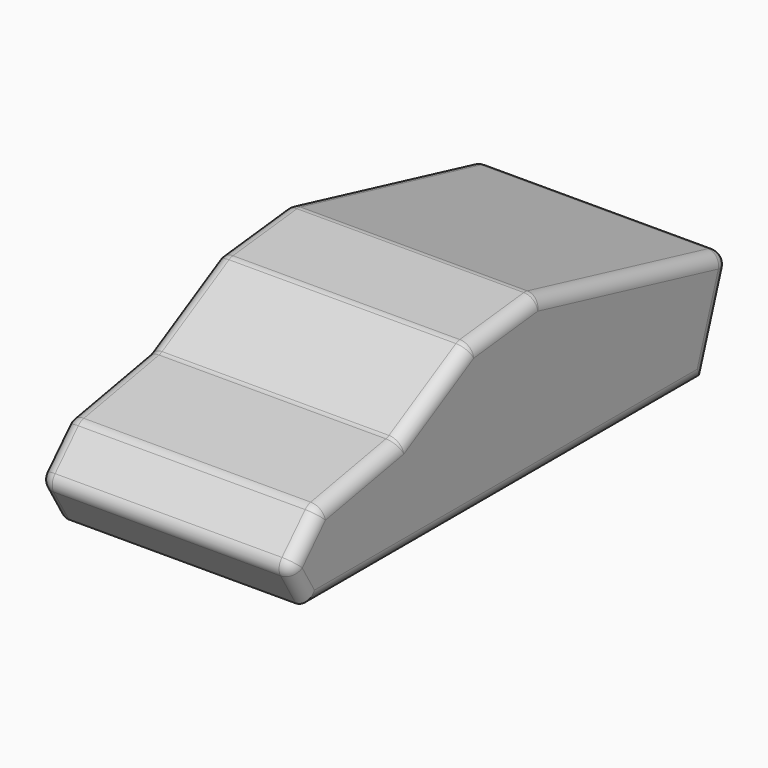
from build123d import *

# Parameters (mm, degrees)
F1_DEPTH     = 99.822
F2_R         = 5.08
F3_R         = 5.08
F4_F1_R      = 5.08
F4_T2_DEPTH  = 89.662
F4_T7_DEPTH  = 5.1816
F4_T13_DEPTH = 5.1816
F4_T19_DEPTH = 5.1816
F4_T25_DEPTH = 5.1816
F4_T31_DEPTH = 5.1816
F4_T37_DEPTH = 5.1816
F4_T43_DEPTH = 5.1816
F4_T49_DEPTH = 5.1816
F4_T55_DEPTH = 5.1816
F4_T61_DEPTH = 5.1816


# Not quite as in the source:
# - a fillet or chamfer that OpenCascade refuses, or shapes differently, is made with other operations: its cross-section is extruded or revolved along the edge and cut away or added


with BuildPart() as f1:
    # F0 (on Right) → F1 (new body)
    with BuildSketch(Plane.YZ):
        Polygon((-82.3224335909, 15.9557517618), (-72.8414729238, 0), (122.7899119258, 0), (136.201992631, 39.3112748861), (40.6987294555, 62.4355487525), (7.1685267612, 58.7356649339), (-27.5178905576, 39.3112748861), (-67.0604035258, 31.9115035236), align=None)
    extrude(amount=F1_DEPTH)

    # F2
    f2_edges = [f1.edges().sort_by_distance(p)[0] for p in [
        (99.822, -47.289147, 35.611389),
        (99.822, -74.691419, 23.933628),
        (99.822, -77.581953, 7.977876),
        (99.822, 24.97422, 0),
        (99.822, 129.495952, 19.655637),
        (99.822, 88.450361, 50.873412),
        (99.822, 23.933628, 60.585607),
        (99.822, -10.174682, 49.02347),
    ]]
    fillet(f2_edges, radius=F2_R)

    # F3
    f3_edges = [f1.edges().sort_by_distance(p)[0] for p in [
        (0, -47.289147, 35.611389),
        (0, -74.691419, 23.933628),
        (0, -77.581953, 7.977876),
        (0, 24.97422, 0),
        (0, 129.495952, 19.655637),
        (0, 88.450361, 50.873412),
        (0, 23.933628, 60.585607),
        (0, -10.174682, 49.02347),
    ]]
    fillet(f3_edges, radius=F3_R)

    # F4: fillet of radius 5.08 on 8 edges, made by hand

    # F4_f1
    f4_f1_edges = [f1.edges().sort_by_distance(p)[0] for p in [
        (49.911, -27.5178905576, 39.3112748861),
        (1.4878975516, -27.0040618743, 37.8937040228),
        (98.3341025696, -27.0040618325, 37.8937039074),
    ]]
    fillet(f4_f1_edges, radius=F4_F1_R)

    # F4_s3 → F4_t2 (cut)
    with BuildSketch(Plane.YZ.offset(5.08)):
        with BuildLine():
            ThreePointArc((-65.453685614, 32.2121759973), (-66.9382582043, 31.6859414336), (-68.1902824988, 30.7302669295))
            Line((-68.1902824988, 30.7302669295), (-68.2637028962, 30.8004951663))
            Line((-68.2637028962, 30.8004951663), (-67.1112263438, 32.0053564923))
            Line((-67.1112263438, 32.0053564923), (-65.4723740737, 32.3120424155))
            Line((-65.4723740737, 32.3120424155), (-65.453685614, 32.2121759973))
        make_face()
        with BuildLine():
            ThreePointArc((-79.6549091873, 18.7445260612), (-81.0311938802, 15.8085415748), (-80.3510820874, 12.6381137788))
            Line((-80.3510820874, 12.6381137788), (-80.4384259429, 12.5862137699))
            Line((-80.4384259429, 12.5862137699), (-82.4492044764, 15.9702045126))
            Line((-82.4492044764, 15.9702045126), (-79.7283295848, 18.8147542979))
            Line((-79.7283295848, 18.8147542979), (-79.6549091873, 18.7445260612))
        make_face()
        with BuildLine():
            ThreePointArc((6.2686920086, 58.2317575672), (7.2001593092, 58.6369802666), (8.1936269176, 58.8487794151))
            Line((8.1936269176, 58.8487794151), (8.1824835206, 58.9497664672))
            Line((8.1824835206, 58.9497664672), (7.1368813611, 58.8343896965))
            Line((7.1368813611, 58.8343896965), (6.2190499134, 58.3204041823))
            Line((6.2190499134, 58.3204041823), (6.2686920086, 58.2317575672))
        make_face()
        with BuildLine():
            ThreePointArc((39.8125749839, 62.3377662065), (40.6937772364, 62.3580687153), (41.5652241428, 62.2257437701))
            Line((41.5652241428, 62.2257437701), (41.589133729, 62.3244903735))
            Line((41.589133729, 62.3244903735), (40.7053091479, 62.5384914556))
            Line((40.7053091479, 62.5384914556), (39.8014315869, 62.4387532586))
            Line((39.8014315869, 62.4387532586), (39.8125749839, 62.3377662065))
        make_face()
        with BuildLine():
            ThreePointArc((130.792336403, 40.6211188431), (134.0495526612, 38.1291725243), (134.4047361425, 34.0434536277))
            Line((134.4047361425, 34.0434536277), (134.5008937235, 34.0106469268))
            Line((134.5008937235, 34.0106469268), (136.3340953417, 39.3838246104))
            Line((136.3340953417, 39.3838246104), (130.8162459892, 40.7198654465))
            Line((130.8162459892, 40.7198654465), (130.792336403, 40.6211188431))
        make_face()
    extrude(amount=F4_T2_DEPTH, mode=Mode.SUBTRACT)


with BuildPart() as f4_tool5:
    # F4_s6 → F4_t7 (new body)
    with BuildSketch(Plane.YZ.offset(5.08)):
        Polygon((129.5968570941, 35.6837886716), (130.8162459892, 40.7198654465), (136.3340953417, 39.3838246104), (134.5008937235, 34.0106469268), align=None)
    extrude(amount=-F4_T7_DEPTH)

    # F4_s8 → F4_t9 (revolve, cut)
    with BuildSketch(Plane(origin=(5.08, 129.5968570941, 35.6837886716), x_dir=(0, -0.8765148754, -0.4813747742), z_dir=(0, 0.4813747742, -0.8765148754))):
        with BuildLine():
            ThreePointArc((0, -5.08), (5.08, 0), (0, 5.08))
            Line((0, 5.08), (0, -5.08))
        make_face()
    revolve(axis=Axis((5.08, 129.5968570941, 35.6837886716), (-1, 0, 0)), mode=Mode.SUBTRACT)


with BuildPart() as f1_1:
    add(f1.part)

    # F4_t4: cut F4_tool5
    add(f4_tool5.part, mode=Mode.SUBTRACT)


with BuildPart() as f4_tool11:
    # F4_s12 → F4_t13 (new body)
    with BuildSketch(Plane.YZ.offset(94.742)):
        Polygon((129.5968570941, 35.6837886716), (130.8162459892, 40.7198654465), (136.3340953417, 39.3838246104), (134.5008937235, 34.0106469268), align=None)
    extrude(amount=F4_T13_DEPTH)

    # F4_s14 → F4_t15 (revolve, cut)
    with BuildSketch(Plane(origin=(94.742, 129.5968570941, 35.6837886716), x_dir=(0, -0.8765148754, -0.4813747742), z_dir=(0, -0.4813747742, 0.8765148754))):
        with BuildLine():
            ThreePointArc((0, -5.08), (5.08, 0), (0, 5.08))
            Line((0, 5.08), (0, -5.08))
        make_face()
    revolve(axis=Axis((94.742, 129.5968570941, 35.6837886716), (1, 0, 0)), mode=Mode.SUBTRACT)


with BuildPart() as f1_2:
    add(f1_1.part)

    # F4_t10: cut F4_tool11
    add(f4_tool11.part, mode=Mode.SUBTRACT)


with BuildPart() as f4_tool17:
    # F4_s18 → F4_t19 (new body)
    with BuildSketch(Plane.YZ.offset(5.08)):
        Polygon((40.369744834, 57.2884135986), (39.8014315869, 62.4387532586), (40.7053091479, 62.5384914556), (41.589133729, 62.3244903735), align=None)
    extrude(amount=-F4_T19_DEPTH)

    # F4_s20 → F4_t21 (revolve, cut)
    with BuildSketch(Plane(origin=(5.08, 40.369744834, 57.2884135986), x_dir=(0, -0.063785906, -0.9979636056), z_dir=(0, 0.9979636056, -0.063785906))):
        with BuildLine():
            ThreePointArc((0, -5.08), (5.08, 0), (0, 5.08))
            Line((0, 5.08), (0, -5.08))
        make_face()
    revolve(axis=Axis((5.08, 40.369744834, 57.2884135986), (-1, 0, 0)), mode=Mode.SUBTRACT)


with BuildPart() as f1_3:
    add(f1_2.part)

    # F4_t16: cut F4_tool17
    add(f4_tool17.part, mode=Mode.SUBTRACT)


with BuildPart() as f4_tool23:
    # F4_s24 → F4_t25 (new body)
    with BuildSketch(Plane.YZ.offset(94.742)):
        Polygon((40.369744834, 57.2884135986), (39.8014315869, 62.4387532586), (40.7053091479, 62.5384914556), (41.589133729, 62.3244903735), align=None)
    extrude(amount=F4_T25_DEPTH)

    # F4_s26 → F4_t27 (revolve, cut)
    with BuildSketch(Plane(origin=(94.742, 40.369744834, 57.2884135986), x_dir=(0, -0.063785906, -0.9979636056), z_dir=(0, -0.9979636056, 0.063785906))):
        with BuildLine():
            ThreePointArc((0, -5.08), (5.08, 0), (0, 5.08))
            Line((0, 5.08), (0, -5.08))
        make_face()
    revolve(axis=Axis((94.742, 40.369744834, 57.2884135986), (1, 0, 0)), mode=Mode.SUBTRACT)


with BuildPart() as f1_4:
    add(f1_3.part)

    # F4_t22: cut F4_tool23
    add(f4_tool23.part, mode=Mode.SUBTRACT)


with BuildPart() as f4_tool29:
    # F4_s30 → F4_t31 (new body)
    with BuildSketch(Plane.YZ.offset(5.08)):
        Polygon((8.7507967676, 53.7994268073), (6.2190499134, 58.3204041823), (7.1368813611, 58.8343896965), (8.1824835206, 58.9497664672), align=None)
    extrude(amount=-F4_T31_DEPTH)

    # F4_s32 → F4_t33 (revolve, cut)
    with BuildSketch(Plane(origin=(5.08, 8.7507967676, 53.7994268073), x_dir=(0, 0.3052435942, -0.952274303), z_dir=(0, 0.952274303, 0.3052435942))):
        with BuildLine():
            ThreePointArc((0, -5.08), (5.08, 0), (0, 5.08))
            Line((0, 5.08), (0, -5.08))
        make_face()
    revolve(axis=Axis((5.08, 8.7507967676, 53.7994268073), (-1, 0, 0)), mode=Mode.SUBTRACT)


with BuildPart() as f1_5:
    add(f1_4.part)

    # F4_t28: cut F4_tool29
    add(f4_tool29.part, mode=Mode.SUBTRACT)


with BuildPart() as f4_tool35:
    # F4_s36 → F4_t37 (new body)
    with BuildSketch(Plane.YZ.offset(94.742)):
        Polygon((8.7507967676, 53.7994268073), (6.2190499134, 58.3204041823), (7.1368813611, 58.8343896965), (8.1824835206, 58.9497664672), align=None)
    extrude(amount=F4_T37_DEPTH)

    # F4_s38 → F4_t39 (revolve, cut)
    with BuildSketch(Plane(origin=(94.742, 8.7507967676, 53.7994268073), x_dir=(0, 0.3052435942, -0.952274303), z_dir=(0, -0.952274303, -0.3052435942))):
        with BuildLine():
            ThreePointArc((0, -5.08), (5.08, 0), (0, 5.08))
            Line((0, 5.08), (0, -5.08))
        make_face()
    revolve(axis=Axis((94.742, 8.7507967676, 53.7994268073), (1, 0, 0)), mode=Mode.SUBTRACT)


with BuildPart() as f1_6:
    add(f1_5.part)

    # F4_t34: cut F4_tool35
    add(f4_tool35.part, mode=Mode.SUBTRACT)


with BuildPart() as f4_tool41:
    # F4_s42 → F4_t43 (new body)
    with BuildSketch(Plane.YZ.offset(5.08)):
        Polygon((-75.9838893162, 15.2331142218), (-79.7283295848, 18.8147542979), (-82.4492044764, 15.9702045126), (-80.4384259429, 12.5862137699), align=None)
    extrude(amount=-F4_T43_DEPTH)

    # F4_s44 → F4_t45 (revolve, cut)
    with BuildSketch(Plane(origin=(5.08, -75.9838893162, 15.2331142218), x_dir=(0, 0.9935638905, -0.113273101), z_dir=(0, 0.113273101, 0.9935638905))):
        with BuildLine():
            ThreePointArc((0, -5.08), (5.08, 0), (0, 5.08))
            Line((0, 5.08), (0, -5.08))
        make_face()
    revolve(axis=Axis((5.08, -75.9838893162, 15.2331142218), (-1, 0, 0)), mode=Mode.SUBTRACT)


with BuildPart() as f1_7:
    add(f1_6.part)

    # F4_t40: cut F4_tool41
    add(f4_tool41.part, mode=Mode.SUBTRACT)


with BuildPart() as f4_tool47:
    # F4_s48 → F4_t49 (new body)
    with BuildSketch(Plane.YZ.offset(94.742)):
        Polygon((-75.9838893162, 15.2331142218), (-79.7283295848, 18.8147542979), (-82.4492044764, 15.9702045126), (-80.4384259429, 12.5862137699), align=None)
    extrude(amount=F4_T49_DEPTH)

    # F4_s50 → F4_t51 (revolve, cut)
    with BuildSketch(Plane(origin=(94.742, -75.9838893162, 15.2331142218), x_dir=(0, 0.9935638905, -0.113273101), z_dir=(0, -0.113273101, -0.9935638905))):
        with BuildLine():
            ThreePointArc((0, -5.08), (5.08, 0), (0, 5.08))
            Line((0, 5.08), (0, -5.08))
        make_face()
    revolve(axis=Axis((94.742, -75.9838893162, 15.2331142218), (1, 0, 0)), mode=Mode.SUBTRACT)


with BuildPart() as f1_8:
    add(f1_7.part)

    # F4_t46: cut F4_tool47
    add(f4_tool47.part, mode=Mode.SUBTRACT)


with BuildPart() as f4_tool53:
    # F4_s54 → F4_t55 (new body)
    with BuildSketch(Plane.YZ.offset(5.08)):
        Polygon((-64.5192626277, 27.2188550901), (-65.4723740737, 32.3120424155), (-67.1112263438, 32.0053564923), (-68.2637028962, 30.8004951663), align=None)
    extrude(amount=-F4_T55_DEPTH)

    # F4_s56 → F4_t57 (revolve, cut)
    with BuildSketch(Plane(origin=(5.08, -64.5192626277, 27.2188550901), x_dir=(0, 0.4761802316, -0.8793477054), z_dir=(0, 0.8793477054, 0.4761802316))):
        with BuildLine():
            ThreePointArc((0, -5.08), (5.08, 0), (0, 5.08))
            Line((0, 5.08), (0, -5.08))
        make_face()
    revolve(axis=Axis((5.08, -64.5192626277, 27.2188550901), (-1, 0, 0)), mode=Mode.SUBTRACT)


with BuildPart() as f1_9:
    add(f1_8.part)

    # F4_t52: cut F4_tool53
    add(f4_tool53.part, mode=Mode.SUBTRACT)


with BuildPart() as f4_tool59:
    # F4_s60 → F4_t61 (new body)
    with BuildSketch(Plane.YZ.offset(94.742)):
        Polygon((-64.5192626277, 27.2188550901), (-65.4723740737, 32.3120424155), (-67.1112263438, 32.0053564923), (-68.2637028962, 30.8004951663), align=None)
    extrude(amount=F4_T61_DEPTH)

    # F4_s62 → F4_t63 (revolve, cut)
    with BuildSketch(Plane(origin=(94.742, -64.5192626277, 27.2188550901), x_dir=(0, 0.4761802316, -0.8793477054), z_dir=(0, -0.8793477054, -0.4761802316))):
        with BuildLine():
            ThreePointArc((0, -5.08), (5.08, 0), (0, 5.08))
            Line((0, 5.08), (0, -5.08))
        make_face()
    revolve(axis=Axis((94.742, -64.5192626277, 27.2188550901), (1, 0, 0)), mode=Mode.SUBTRACT)


with BuildPart() as f1_10:
    add(f1_9.part)

    # F4_t58: cut F4_tool59
    add(f4_tool59.part, mode=Mode.SUBTRACT)


solid = f1_10.part
